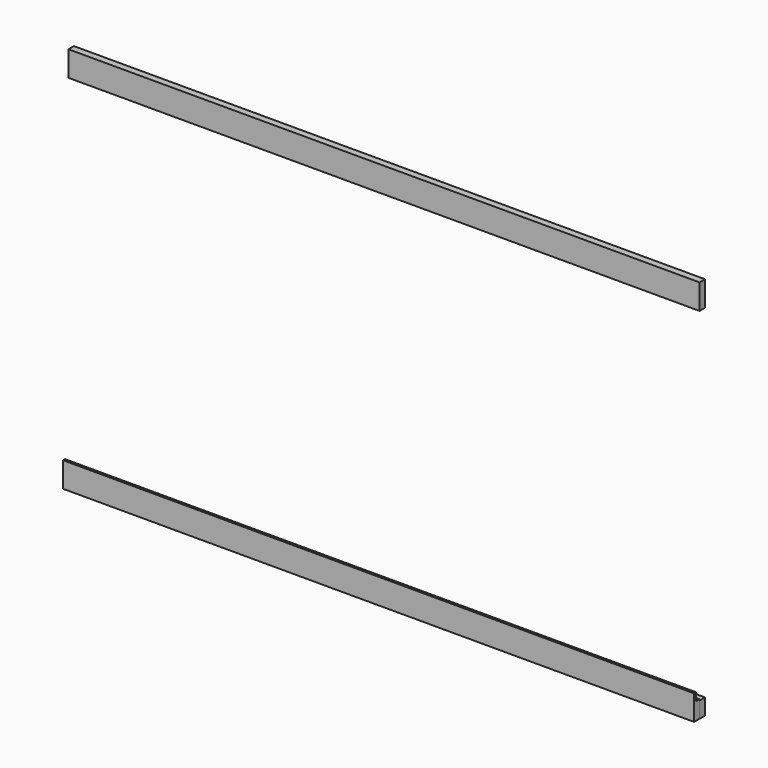
from build123d import *

# Parameters (mm, degrees)
F0_W     = 3505.2
F0_H     = 139.7
F1_DEPTH = 38.1
F0_H_2   = 88.9
F2_W     = 38.1
F2_H     = 139.7
F3_DEPTH = 3505.2
F4_W     = 62.6018452736
F4_H     = 44.45
F5_DEPTH = 3505.2


# Not quite as in the source:
# - a feature names something its author has since deleted; it is built from what else it names


with BuildPart() as f1:
    # F0 (on Front) → F1 (new body)
    with BuildSketch(Plane.XZ):
        with Locations((1752.6, -69.85)):
            Rectangle(F0_W, F0_H)
    extrude(amount=F1_DEPTH)


with BuildPart() as f1b:
    # F0 (on Front) → F1, piece 2 (new body)
    with BuildSketch(Plane.XZ):
        with Locations((1752.6, -2089.15)):
            Rectangle(F0_W, F0_H_2)
    extrude(amount=F1_DEPTH)


with BuildPart() as f3:
    # F2 (on face) → F3 (new body, through all)
    with BuildSketch(Plane(origin=(0, 0, 0), x_dir=(0, -1, 0), z_dir=(-1, 0, 0))):
        with Locations((57.15, -2063.75)):
            Rectangle(F2_W, F2_H)
    extrude(amount=-F3_DEPTH)

    # F4 (on face) → F5 (cut, through all)
    with BuildSketch(Plane(origin=(0, 0, 0), x_dir=(0, -1, 0), z_dir=(-1, 0, 0))):
        with Locations((31.3009226368, -2016.125)):
            Rectangle(F4_W, F4_H)
    extrude(amount=-F5_DEPTH, mode=Mode.SUBTRACT)


solid = Compound([f1.part, f1b.part, f3.part])
